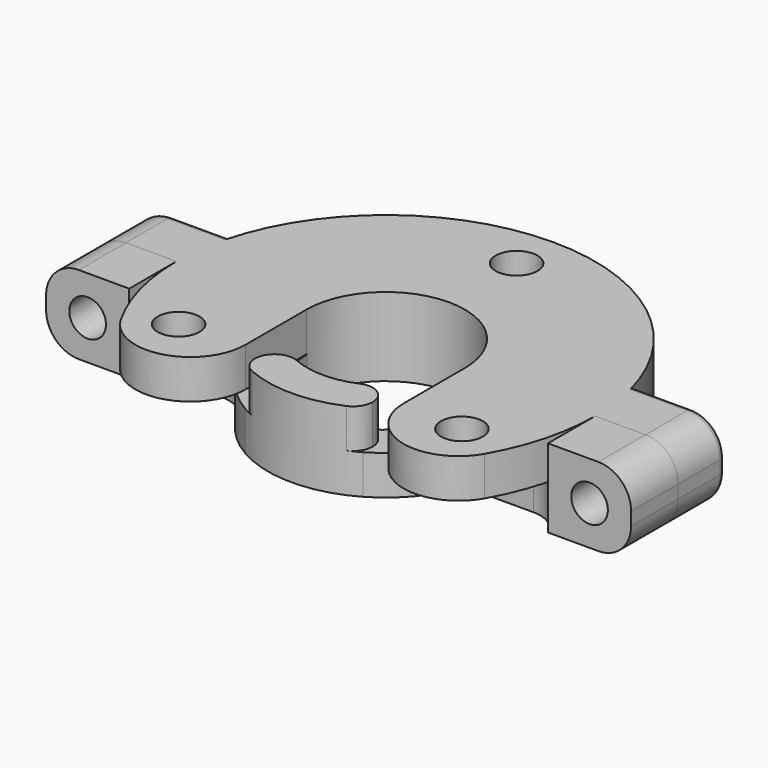
from build123d import *

# Parameters (mm, degrees)
F0_R          = 1.6
F1_DEPTH      = 3
F2_DEPTH      = 3
F3_R          = 1.4
F4_DEPTH      = 16.001
F5_R          = 2.5
F6_R          = 0.5
F7_R          = 4.2
F9_DEPTH      = 3
F10_DEPTH     = 3
F11_R         = 1.4
F12_DEPTH     = 25
F13_T1_DEPTH  = 3
F13_T3_DEPTH  = 3
F13_T5_DEPTH  = 3
F13_T7_DEPTH  = 3
F13_T9_DEPTH  = 17
F13_T11_DEPTH = 17
F13_T13_DEPTH = 17
F13_T15_DEPTH = 17
F14_T1_DEPTH  = 10.2630914396
F14_T3_DEPTH  = 5.5205236091


# Not quite as in the source:
# - a fillet or chamfer that OpenCascade refuses, or shapes differently, is made with other operations: its cross-section is extruded or revolved along the edge and cut away or added


with BuildPart() as f1:
    # F0 (on Top) → F1 (new body)
    with BuildSketch(Plane.XY):
        with BuildLine():
            ThreePointArc((-16, 0), (-15.8377151213, 2.273055155), (-15.3541525328, 4.5))
            Line((-15.3541525328, 4.5), (-22.3541525328, 4.5))
            Line((-22.3541525328, 4.5), (-22.3541525328, 0))
            Line((-22.3541525328, 0), (-16, 0))
        make_face()
        with BuildLine():
            Line((7.65, 0), (16, 0))
            ThreePointArc((16, 0), (15.8377151213, 2.273055155), (15.3541525328, 4.5))
            ThreePointArc((15.3541525328, 4.5), (0, 16), (-15.3541525328, 4.5))
            ThreePointArc((-15.3541525328, 4.5), (-15.8377151213, 2.273055155), (-16, 0))
            Line((-16, 0), (-7.65, 0))
            ThreePointArc((-7.65, 0), (0, 7.65), (7.65, 0))
        make_face()
        with Locations((0, 12.5)):
            Circle(F0_R, mode=Mode.SUBTRACT)
        with BuildLine():
            ThreePointArc((-6.05, 0), (0, 6.05), (6.05, 0))
            Line((6.05, 0), (7.65, 0))
            ThreePointArc((7.65, 0), (0, 7.65), (-7.65, 0))
            Line((-7.65, 0), (-6.05, 0))
        make_face()
        with BuildLine():
            ThreePointArc((15.3541525328, 4.5), (15.8377151213, 2.273055155), (16, 0))
            Line((16, 0), (22.3541525328, 0))
            Line((22.3541525328, 0), (22.3541525328, 4.5))
            Line((22.3541525328, 4.5), (15.3541525328, 4.5))
        make_face()
        with BuildLine():
            Line((-6.05, -14.8120727786), (-6.05, 0))
            Line((-6.05, 0), (-7.65, 0))
            Line((-7.65, 0), (-16, 0))
            ThreePointArc((-16, 0), (-13.2815661727, -8.9218832093), (-6.05, -14.8120727786))
        make_face()
        with Locations((-10.8253175473, -6.25)):
            Circle(F0_R, mode=Mode.SUBTRACT)
        with BuildLine():
            Line((6.05, 0), (6.05, -14.8120727786))
            ThreePointArc((6.05, -14.8120727786), (13.2815661727, -8.9218832093), (16, 0))
            Line((16, 0), (7.65, 0))
            Line((7.65, 0), (6.05, 0))
        make_face()
        with Locations((10.8253175473, -6.25)):
            Circle(F0_R, mode=Mode.SUBTRACT)
    extrude(amount=F1_DEPTH)

    # F0 (on Top) → F2 (join)
    with BuildSketch(Plane.XY):
        with BuildLine():
            Line((7.65, 0), (16, 0))
            ThreePointArc((16, 0), (15.8377151213, 2.273055155), (15.3541525328, 4.5))
            ThreePointArc((15.3541525328, 4.5), (0, 16), (-15.3541525328, 4.5))
            ThreePointArc((-15.3541525328, 4.5), (-15.8377151213, 2.273055155), (-16, 0))
            Line((-16, 0), (-7.65, 0))
            ThreePointArc((-7.65, 0), (0, 7.65), (7.65, 0))
        make_face()
        with Locations((0, 12.5)):
            Circle(F0_R, mode=Mode.SUBTRACT)
        with BuildLine():
            ThreePointArc((-6.05, 0), (0, 6.05), (6.05, 0))
            Line((6.05, 0), (7.65, 0))
            ThreePointArc((7.65, 0), (0, 7.65), (-7.65, 0))
            Line((-7.65, 0), (-6.05, 0))
        make_face()
        with BuildLine():
            ThreePointArc((15.3541525328, 4.5), (15.8377151213, 2.273055155), (16, 0))
            Line((16, 0), (22.3541525328, 0))
            Line((22.3541525328, 0), (22.3541525328, 4.5))
            Line((22.3541525328, 4.5), (15.3541525328, 4.5))
        make_face()
        with BuildLine():
            ThreePointArc((-16, 0), (-15.8377151213, 2.273055155), (-15.3541525328, 4.5))
            Line((-15.3541525328, 4.5), (-22.3541525328, 4.5))
            Line((-22.3541525328, 4.5), (-22.3541525328, 0))
            Line((-22.3541525328, 0), (-16, 0))
        make_face()
    extrude(amount=-F2_DEPTH)

    # F3 (on face) → F4 (cut, through all)
    with BuildSketch(Plane.XZ):
        with Locations((19.1770762664, 0)):
            Circle(F3_R)
        with Locations((-19.1770762664, 0)):
            Circle(F3_R)
    extrude(amount=-F4_DEPTH, mode=Mode.SUBTRACT)

    # F5
    f5_edges = [f1.edges().sort_by_distance(p)[0] for p in [
        (-22.354153, 2.25, 3),
        (22.354153, 2.25, 3),
        (-22.354153, 2.25, -3),
        (22.354153, 2.25, -3),
    ]]
    fillet(f5_edges, radius=F5_R)

    # F6
    f6_edges = [f1.edges().sort_by_distance(p)[0] for p in [
        (-17.604153, 4.5, 3),
        (17.604153, 4.5, 3),
        (-21.621919, 4.5, 2.267767),
        (-22.354153, 4.5, 0),
        (-17.604153, 4.5, -3),
        (-21.621919, 4.5, -2.267767),
        (17.604153, 4.5, -3),
        (22.354153, 4.5, 0),
        (21.621919, 4.5, 2.267767),
        (21.621919, 4.5, -2.267767),
    ]]
    fillet(f6_edges, radius=F6_R)

    # F7
    f7_edges = [f1.edges().sort_by_distance(p)[0] for p in [
        (-6.05, -14.812073, 1.5),
        (6.05, -14.812073, 1.5),
    ]]
    fillet(f7_edges, radius=F7_R)


with BuildPart() as f9:
    # F8 (on Top) → F9 (new body)
    with BuildSketch(Plane.XY):
        with BuildLine():
            ThreePointArc((-4.5, -3.9686269666), (-5.6124860802, -2.1213203436), (-6, 0))
            Line((-6, 0), (-9, 0))
            ThreePointArc((-9, 0), (-8.8703870369, -1.5219178085), (-8.4852813742, -3))
            ThreePointArc((-8.4852813742, -3), (-6.9210216111, -5.7532130031), (-4.5, -7.7942286341))
            Line((-4.5, -7.7942286341), (-4.5, -3.9686269666))
        make_face()
        with BuildLine():
            ThreePointArc((4.5, -3.9686269666), (0, -6), (-4.5, -3.9686269666))
            Line((-4.5, -3.9686269666), (-4.5, -7.7942286341))
            ThreePointArc((-4.5, -7.7942286341), (0, -9), (4.5, -7.7942286341))
            Line((4.5, -7.7942286341), (4.5, -3.9686269666))
        make_face()
        with BuildLine():
            ThreePointArc((-8.4852813742, -3), (-8.8703870369, -1.5219178085), (-9, 0))
            Line((-9, 0), (-16, 0))
            Line((-16, 0), (-16, -3))
            Line((-16, -3), (-8.4852813742, -3))
        make_face()
        with BuildLine():
            ThreePointArc((6, 0), (5.6124860802, -2.1213203436), (4.5, -3.9686269666))
            Line((4.5, -3.9686269666), (4.5, -7.7942286341))
            ThreePointArc((4.5, -7.7942286341), (6.9210216111, -5.7532130031), (8.4852813742, -3))
            ThreePointArc((8.4852813742, -3), (8.8703870369, -1.5219178085), (9, 0))
            Line((9, 0), (6, 0))
        make_face()
        Polygon((-16, -3), (-16, 0), (-22.3541525328, 0), (-22.3541525328, -4.5), (-16, -4.5), align=None)
        with BuildLine():
            Line((16, 0), (9, 0))
            ThreePointArc((9, 0), (8.8703870369, -1.5219178085), (8.4852813742, -3))
            Line((8.4852813742, -3), (16, -3))
            Line((16, -3), (16, 0))
        make_face()
        Polygon((22.3541525328, 0), (16, 0), (16, -3), (16, -4.5), (22.3541525328, -4.5), align=None)
    extrude(amount=-F9_DEPTH)

    # F8 (on Top) → F10 (join)
    with BuildSketch(Plane.XY):
        Polygon((-16, -3), (-16, 0), (-22.3541525328, 0), (-22.3541525328, -4.5), (-16, -4.5), align=None)
        Polygon((22.3541525328, 0), (16, 0), (16, -3), (16, -4.5), (22.3541525328, -4.5), align=None)
        with BuildLine():
            ThreePointArc((4.5, -3.9686269666), (0, -6), (-4.5, -3.9686269666))
            Line((-4.5, -3.9686269666), (-4.5, -7.7942286341))
            ThreePointArc((-4.5, -7.7942286341), (0, -9), (4.5, -7.7942286341))
            Line((4.5, -7.7942286341), (4.5, -3.9686269666))
        make_face()
    extrude(amount=F10_DEPTH)

    # F11 (on face) → F12 (cut)
    with BuildSketch(Plane.XZ.offset(4.5)):
        with Locations((-19.1770762664, 0)):
            Circle(F11_R)
        with Locations((19.1770762664, 0)):
            Circle(F11_R)
    extrude(amount=-F12_DEPTH, mode=Mode.SUBTRACT)

    # F13: fillet of radius 2.5 on 8 edges, made by hand

    # F13_s2 → F13_t1 (join)
    with BuildSketch(Plane.XY.offset(-3)):
        with BuildLine():
            ThreePointArc((-16, -4.5), (-15.0780185463, -3.4083499337), (-13.7087121525, -3))
            Line((-13.7087121525, -3), (-16, -3))
            Line((-16, -3), (-16, -4.5))
        make_face()
    extrude(amount=F13_T1_DEPTH)

    # F13_s4 → F13_t3 (join)
    with BuildSketch(Plane.XY.offset(-3)):
        with BuildLine():
            ThreePointArc((-10.0995049384, -3), (-8.8226201422, -3.3506826159), (-7.9039603865, -4.3043478261))
            ThreePointArc((-7.9039603865, -4.3043478261), (-8.220531746, -3.6637218527), (-8.4852813742, -3))
            Line((-8.4852813742, -3), (-10.0995049384, -3))
        make_face()
    extrude(amount=F13_T3_DEPTH)

    # F13_s6 → F13_t5 (join)
    with BuildSketch(Plane.XY.offset(-3)):
        with BuildLine():
            ThreePointArc((7.9039603865, -4.3043478261), (8.8226201422, -3.3506826159), (10.0995049384, -3))
            Line((10.0995049384, -3), (8.4852813742, -3))
            ThreePointArc((8.4852813742, -3), (8.220531746, -3.6637218527), (7.9039603865, -4.3043478261))
        make_face()
    extrude(amount=F13_T5_DEPTH)

    # F13_s8 → F13_t7 (join)
    with BuildSketch(Plane.XY.offset(-3)):
        with BuildLine():
            ThreePointArc((13.7087121525, -3), (15.0780185463, -3.4083499337), (16, -4.5))
            Line((16, -4.5), (16, -3))
            Line((16, -3), (13.7087121525, -3))
        make_face()
    extrude(amount=F13_T7_DEPTH)

    # F13_s10 → F13_t9 (cut)
    with BuildSketch(Plane.XZ.offset(-6.25)):
        with BuildLine():
            ThreePointArc((-22.3541525328, -0.5), (-21.6219194858, -2.267766953), (-19.8541525328, -3))
            Line((-19.8541525328, -3), (-22.3541525328, -3))
            Line((-22.3541525328, -3), (-22.3541525328, -0.5))
        make_face()
    extrude(amount=F13_T9_DEPTH, mode=Mode.SUBTRACT)

    # F13_s12 → F13_t11 (cut)
    with BuildSketch(Plane.XZ.offset(-6.25)):
        with BuildLine():
            ThreePointArc((19.8541525328, -3), (21.6219194858, -2.267766953), (22.3541525328, -0.5))
            Line((22.3541525328, -0.5), (22.3541525328, -3))
            Line((22.3541525328, -3), (19.8541525328, -3))
        make_face()
    extrude(amount=F13_T11_DEPTH, mode=Mode.SUBTRACT)

    # F13_s14 → F13_t13 (cut)
    with BuildSketch(Plane.XZ.offset(-6.25)):
        with BuildLine():
            ThreePointArc((-19.8541525328, 3), (-21.6219194858, 2.267766953), (-22.3541525328, 0.5))
            Line((-22.3541525328, 0.5), (-22.3541525328, 3))
            Line((-22.3541525328, 3), (-19.8541525328, 3))
        make_face()
    extrude(amount=F13_T13_DEPTH, mode=Mode.SUBTRACT)

    # F13_s16 → F13_t15 (cut)
    with BuildSketch(Plane.XZ.offset(-6.25)):
        with BuildLine():
            ThreePointArc((22.3541525328, 0.5), (21.6219194858, 2.267766953), (19.8541525328, 3))
            Line((19.8541525328, 3), (22.3541525328, 3))
            Line((22.3541525328, 3), (22.3541525328, 0.5))
        make_face()
    extrude(amount=F13_T15_DEPTH, mode=Mode.SUBTRACT)

    # F14: fillet of radius 1.5 on 4 edges, made by hand

    # F14_s2 → F14_t1 (cut)
    with BuildSketch(Plane.XY):
        with BuildLine():
            ThreePointArc((-2.4, -5.4990908339), (-3.8215838363, -5.6188735026), (-4.5, -6.8738635424))
            Line((-4.5, -6.8738635424), (-4.5, -3.9686269666))
            ThreePointArc((-4.5, -3.9686269666), (-3.5338477489, -4.8489091647), (-2.4, -5.4990908339))
        make_face()
        with BuildLine():
            ThreePointArc((2.4, -5.4990908339), (3.8215838363, -5.6188735026), (4.5, -6.8738635424))
            Line((4.5, -6.8738635424), (4.5, -3.9686269666))
            ThreePointArc((4.5, -3.9686269666), (3.5338477489, -4.8489091647), (2.4, -5.4990908339))
        make_face()
    extrude(amount=F14_T1_DEPTH, mode=Mode.SUBTRACT)

    # F14_s4 → F14_t3 (cut)
    with BuildSketch(Plane.XY):
        with BuildLine():
            ThreePointArc((-3.6, -8.2486362509), (-4.2549900398, -7.6954473787), (-4.5, -6.8738635424))
            Line((-4.5, -6.8738635424), (-4.5, -7.7942286341))
            ThreePointArc((-4.5, -7.7942286341), (-4.056368027, -8.0340449606), (-3.6, -8.2486362509))
        make_face()
        with BuildLine():
            ThreePointArc((3.6, -8.2486362509), (4.2549900398, -7.6954473787), (4.5, -6.8738635424))
            Line((4.5, -6.8738635424), (4.5, -7.7942286341))
            ThreePointArc((4.5, -7.7942286341), (4.056368027, -8.0340449606), (3.6, -8.2486362509))
        make_face()
    extrude(amount=F14_T3_DEPTH, mode=Mode.SUBTRACT)


solid = Compound([f1.part, f9.part])
